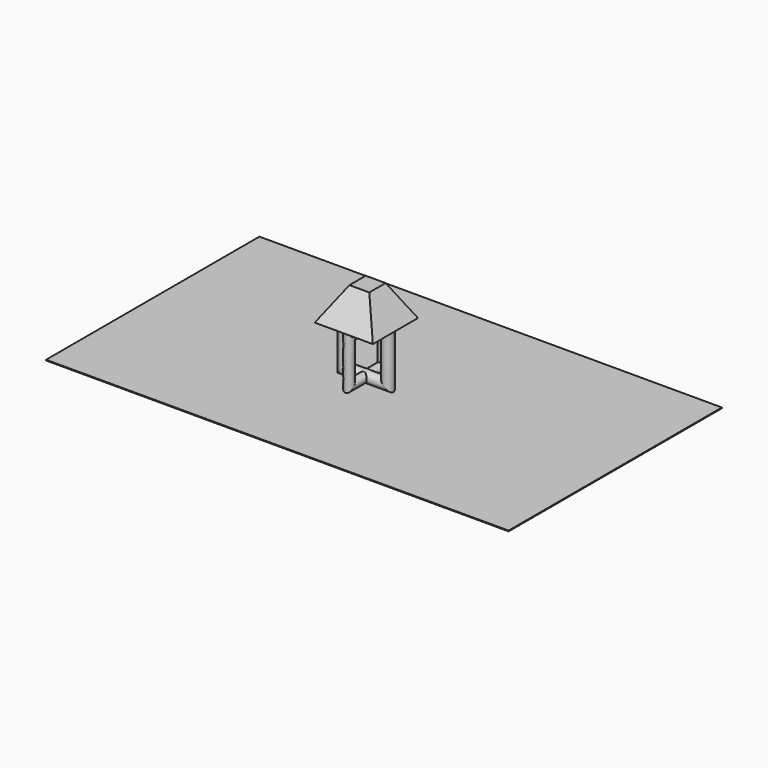
from build123d import *

# Parameters (mm, degrees)
F0_R      = 18.9967095852
F3_R      = 16.2075370321
F9_W      = 69.0684448928
F9_H      = 70.9578543901
F7_W      = 202.4621709585
F7_H      = 196.343092515
F12_W     = 1610.5197668076
F12_H     = 928.3697903156
F13_DEPTH = 2.5


with BuildPart() as f2:
    # F2: sweep along a path in F1
    with BuildLine(Plane.XZ) as f2_path:
        Line((-75.0986859202, 0), (-75.0986859202, 75.1233547926))
        Line((-75.0986859202, 75.1233547926), (74.9753341079, 75.1233547926))
        Line((74.9753341079, 75.1233547926), (74.9753341079, -74.9506577849))
        Line((74.9753341079, -74.9506577849), (-75.0986859202, -74.9506577849))
        Line((-75.0986859202, -74.9506577849), (-75.0986859202, 0))
    # F0 (on Top) → F2 (sweep)
    with BuildSketch(Plane.XY):
        with Locations((-75.2960518003, 0)):
            Circle(F0_R)
    sweep(path=f2_path.line, transition=Transition.RIGHT)

    # F5: sweep along a path in F4
    with BuildLine(Plane.YZ) as f5_path:
        Line((75.5154266953, 75.3782242537), (-74.8513415456, 75.3782242537))
        Line((-74.8513415456, 75.3782242537), (-74.8513415456, -74.7715607285))
        Line((-74.8513415456, -74.7715607285), (74.8644843698, -74.7715607285))
        Line((74.8644843698, -74.7715607285), (75.5154266953, 0))
        Line((75.5154266953, 0), (75.5154266953, 75.3782242537))
    # F3 (on Top) → F5 (sweep)
    with BuildSketch(Plane.XY):
        with Locations((0, 75.2960518003)):
            Circle(F3_R)
    sweep(path=f5_path.line, transition=Transition.RIGHT)


with BuildPart() as f10:
    # F9 (on offset) → F10 section 0
    with BuildSketch(Plane.XY.offset(201)):
        with Locations((-3.7355283275, 9.9890269339)):
            Rectangle(F9_W, F9_H)
    # F7 (on offset) → F10 section 1
    with BuildSketch(Plane.XY.offset(95)):
        with Locations((-0.0616759062, 0.3320425749)):
            Rectangle(F7_W, F7_H)
    loft()


with BuildPart() as f13:
    # F12 (on offset) → F13 (new body)
    with BuildSketch(Plane.XY.offset(-100)):
        with Locations((36.1075997353, 31.9317132235)):
            Rectangle(F12_W, F12_H)
    extrude(amount=-F13_DEPTH)


solid = Compound([f2.part, f10.part, f13.part])
